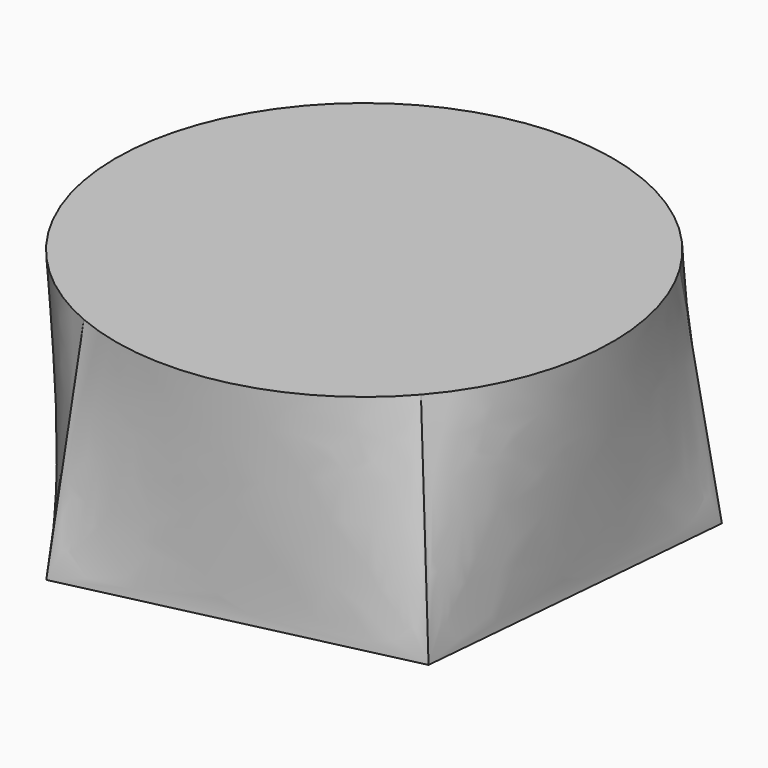
from build123d import *


# Not quite as in the source:
# - the arcs of a loft's sections are written as splines that run evenly, so that the points pair up as in the source's solid


with BuildPart() as f3:
    # F2 (on offset) → F3 section 0
    with BuildSketch(Plane.XY.offset(50.8)):
        with BuildLine():
            add(Edge.make_bspline(
                [(-56.9261720001, 5.0530625782), (-57.190749738, 2.0724151823), (-57.2207451344, -0.9290245136), (-56.8108338665, -6.8997040281), (-56.3709313566, -9.8688833346), (-55.0320467208, -15.7019296265), (-54.1330781644, -18.5657374948), (-51.898187944, -24.1175216058), (-50.5622889304, -26.8054415818), (-47.4864235398, -31.9392601616), (-45.7464883364, -34.3851067349), (-41.9053857897, -38.974548132), (-39.8042573756, -41.1180964425), (-35.2924983654, -45.0501533783), (-32.8819134954, -46.8386221526), (-27.8105925023, -50.0164743355), (-25.1499077762, -51.4058255369), (-22.3969026649, -52.5785246181)],
                knots=[0, 0, 0, 0, 0.125, 0.125, 0.25, 0.25, 0.375, 0.375, 0.5, 0.5, 0.625, 0.625, 0.75, 0.75, 0.875, 0.875, 1, 1, 1, 1], degree=3))
            add(Edge.make_bspline(
                [(-22.3969026649, -52.5785246181), (-19.6438975537, -53.7512236994), (-16.7986278598, -54.7072468902), (-10.9935046529, -56.1624395457), (-8.033709974, -56.6615942622), (-2.0724151823, -57.190749738), (0.9290245136, -57.2207451344), (6.8997040281, -56.8108338665), (9.8688833346, -56.3709313566), (15.7019296265, -55.0320467208), (18.5657374948, -54.1330781644), (24.1175216058, -51.898187944), (26.8054415818, -50.5622889304), (31.9392601616, -47.4864235398), (34.3851067349, -45.7464883364), (38.974548132, -41.9053857897), (41.1180964425, -39.8042573756), (43.0841249104, -37.5483778705)],
                knots=[0, 0, 0, 0, 0.125, 0.125, 0.25, 0.25, 0.375, 0.375, 0.5, 0.5, 0.625, 0.625, 0.75, 0.75, 0.875, 0.875, 1, 1, 1, 1], degree=3))
            add(Edge.make_bspline(
                [(43.0841249104, -37.5483778705), (45.0501533783, -35.2924983654), (46.8386221526, -32.8819134954), (50.0164743355, -27.8105925023), (51.4058255369, -25.1499077762), (53.7512236994, -19.6438975537), (54.7072468902, -16.7986278598), (56.1624395457, -10.9935046529), (56.6615942622, -8.033709974), (57.190749738, -2.0724151823), (57.2207451344, 0.9290245136), (56.8108338665, 6.8997040281), (56.3709313566, 9.8688833346), (55.0320467208, 15.7019296265), (54.1330781644, 18.5657374948), (51.898187944, 24.1175216058), (50.5622889304, 26.8054415818), (49.0243562351, 29.3723508717)],
                knots=[0, 0, 0, 0, 0.125, 0.125, 0.25, 0.25, 0.375, 0.375, 0.5, 0.5, 0.625, 0.625, 0.75, 0.75, 0.875, 0.875, 1, 1, 1, 1], degree=3))
            add(Edge.make_bspline(
                [(49.0243562351, 29.3723508717), (47.4864235398, 31.9392601616), (45.7464883364, 34.3851067349), (41.9053857897, 38.974548132), (39.8042573756, 41.1180964425), (35.2924983654, 45.0501533783), (32.8819134954, 46.8386221526), (27.8105925023, 50.0164743355), (25.1499077762, 51.4058255369), (19.6438975537, 53.7512236994), (16.7986278598, 54.7072468902), (10.9935046529, 56.1624395457), (8.033709974, 56.6615942622), (2.0724151823, 57.190749738), (-0.9290245136, 57.2207451344), (-6.8997040281, 56.8108338665), (-9.8688833346, 56.3709313566), (-12.7854064805, 55.7014890387)],
                knots=[0, 0, 0, 0, 0.125, 0.125, 0.25, 0.25, 0.375, 0.375, 0.5, 0.5, 0.625, 0.625, 0.75, 0.75, 0.875, 0.875, 1, 1, 1, 1], degree=3))
            add(Edge.make_bspline(
                [(-12.7854064805, 55.7014890387), (-15.7019296265, 55.0320467208), (-18.5657374948, 54.1330781644), (-24.1175216058, 51.898187944), (-26.8054415818, 50.5622889304), (-31.9392601616, 47.4864235398), (-34.3851067349, 45.7464883364), (-38.974548132, 41.9053857897), (-41.1180964425, 39.8042573756), (-45.0501533783, 35.2924983654), (-46.8386221526, 32.8819134954), (-50.0164743355, 27.8105925023), (-51.4058255369, 25.1499077762), (-53.7512236994, 19.6438975537), (-54.7072468902, 16.7986278598), (-56.1624395457, 10.9935046529), (-56.6615942622, 8.033709974), (-56.9261720001, 5.0530625782)],
                knots=[0, 0, 0, 0, 0.125, 0.125, 0.25, 0.25, 0.375, 0.375, 0.5, 0.5, 0.625, 0.625, 0.75, 0.75, 0.875, 0.875, 1, 1, 1, 1], degree=3))
        make_face()
    # F0 (on Top) → F3 section 1
    with BuildSketch(Plane.XY):
        Polygon((-64.5657256377, 5.7311890224), (-25.402591142, -59.6346192911), (48.8660609096, -42.5874106504), (55.6034776805, 33.3141520163), (-14.5012218103, 63.1766889029), align=None)
    loft(ruled=True)


solid = f3.part
